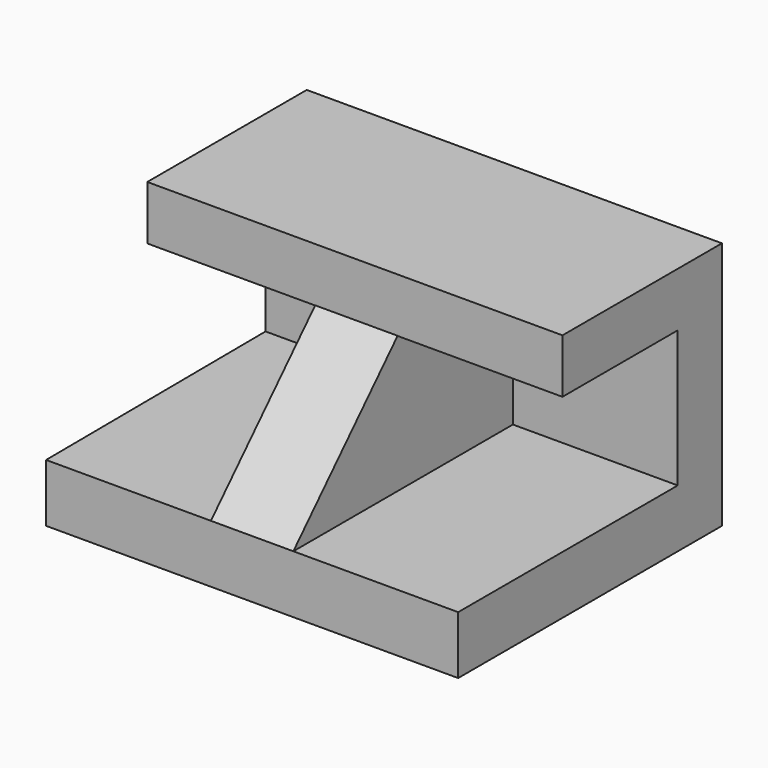
from build123d import *

# Parameters (mm, degrees)
F0_W      = 96.990541555
F0_H      = 38.3299775422
F1_DEPTH  = 50.8
F3_DEPTH  = 101.6
F5_DEPTH  = 25.4
F7_DEPTH  = 38.1
F8_DEPTH  = 38.1
F9_W      = 33.0152064562
F9_H      = 8.3422744647
F10_DEPTH = 47.752
F11_DEPTH = 25.4
F13_DEPTH = 25.4
F15_DEPTH = 63.5
F17_DEPTH = 25.4
F19_DEPTH = 25.4
F20_DEPTH = 9.906
F22_DEPTH = 25.4


# Not quite as in the source:
# - a feature of the source that left no trace in its solid (it failed there, or was rolled back) is left out


with BuildPart() as f1:
    # F0 (on Front) → F1 (new body)
    with BuildSketch(Plane.XZ):
        with Locations((-52.56479932, -19.1649887711)):
            Rectangle(F0_W, F0_H)
    extrude(amount=F1_DEPTH)

    # F2 (on face) → F3 (cut)
    with BuildSketch(Plane.YZ.offset(-4.0695285425)):
        Polygon((-50.8, 0), (-50.8, -29.3875597417), (-30.714739114, -8.3422744647), (-30.714739114, 0), align=None)
    extrude(amount=-F3_DEPTH, mode=Mode.SUBTRACT)

    # F4 (on face) → F5 (cut)
    with BuildSketch(Plane.YZ.offset(-4.0695285425)):
        Polygon((-8.5318721831, -8.3422744647), (-30.714739114, -8.3422744647), (-50.8, -29.3875597417), (-8.5318721831, -29.3875597417), align=None)
    extrude(amount=-F5_DEPTH, mode=Mode.SUBTRACT)

    # F6 (on face) → F7 (cut)
    with BuildSketch(Plane(origin=(-101.0600700974, 0, 0), x_dir=(0, -1, 0), z_dir=(-1, 0, 0))):
        Polygon((50.8, -29.3875597417), (30.714739114, -8.3422744647), (10.0486502051, -8.3422744647), (10.0486502051, -29.3875597417), align=None)
    extrude(amount=-F7_DEPTH, mode=Mode.SUBTRACT)

    # F8 (cut): a face of the model
    f8_faces = [f1.faces().sort_by_distance(p)[0] for p in [
        (-29.4695285425, -25.1662286777, -19.9579957719),
    ]]
    extrude(f8_faces, amount=-F8_DEPTH, mode=Mode.SUBTRACT)

    # F9 (on face) → F10 (cut)
    with BuildSketch(Plane.XZ.offset(30.714739114)):
        with Locations((-84.5524668694, -4.1711372323)):
            Rectangle(F9_W, F9_H)
    extrude(amount=-F10_DEPTH, mode=Mode.SUBTRACT)

    # F11 (cut): a face of the model
    f11_faces = [f1.faces().sort_by_distance(p)[0] for p in [
        (-84.31479932, -10.0486502051, -18.8649171032),
    ]]
    extrude(f11_faces, amount=-F11_DEPTH, mode=Mode.SUBTRACT)

    # F12 (on face) → F13 (cut)
    with BuildSketch(Plane.XY.offset(-29.3875597417)):
        Polygon((-67.5695285425, -50.8), (-67.5695285425, -8.5318721831), (-67.5695285425, 0), (-101.0600700974, 0), (-101.0600700974, -50.8), align=None)
    extrude(amount=-F13_DEPTH, mode=Mode.SUBTRACT)

    # F14 (on face) → F15 (join)
    with BuildSketch(Plane(origin=(-67.5695285425, 0, 0), x_dir=(0, -1, 0), z_dir=(-1, 0, 0))):
        Polygon((50.8, -29.3875597417), (8.5318721831, -8.3422744647), (8.5318721831, -29.3875597417), align=None)
    extrude(amount=-F15_DEPTH)

    # F16 (on face) → F17 (cut)
    with BuildSketch(Plane.YZ.offset(-4.0695285425)):
        Polygon((-8.5318721831, -8.3422744647), (-50.8, -29.3875597417), (-8.5095763206, -29.3875597417), align=None)
    extrude(amount=-F17_DEPTH, mode=Mode.SUBTRACT)

    # F18 (on face) → F19 (cut)
    with BuildSketch(Plane(origin=(-67.5695285425, 0, 0), x_dir=(0, -1, 0), z_dir=(-1, 0, 0))):
        Polygon((50.8, -29.3875597417), (8.5318721831, -8.3422744647), (8.5318721831, -29.1403066367), align=None)
    extrude(amount=-F19_DEPTH, mode=Mode.SUBTRACT)

    # F20 (add): a face of the model
    f20_faces = [f1.faces().sort_by_distance(p)[0] for p in [
        (-35.8195285425, -29.6659360915, -18.8649171032),
    ]]
    extrude(f20_faces, amount=F20_DEPTH)

    # F21 (on face) → F22 (cut)
    with BuildSketch(Plane.YZ.offset(-29.4695285425)):
        Polygon((-55.2151913765, -20.5199263986), (-50.8, -29.3875597417), (-30.714739114, -8.3211602381), align=None)
        Polygon((-12.9470635596, 0.5253588785), (-14.0022137243, 0), (-12.6854875674, 0), align=None)
    extrude(amount=-F22_DEPTH, mode=Mode.SUBTRACT)


solid = f1.part
